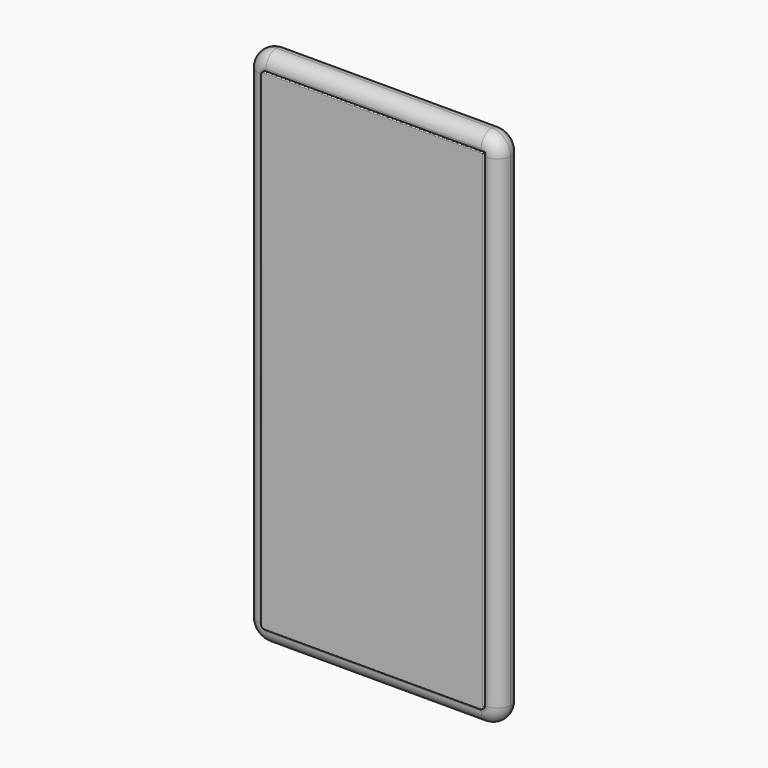
from build123d import *

# Parameters (mm, degrees)
F0_W     = 67
F0_H     = 138
F1_DEPTH = 6.9
F2_R     = 5
F3_R     = 3.44999
F6_DEPTH = 0.5
F7_R     = 0.25


# Not quite as in the source:
# - a fillet or chamfer is up to 0.001 mm smaller than in the source, because OpenCascade refuses the exact size


with BuildPart() as f1:
    # F0 (on Front) → F1 (new body)
    with BuildSketch(Plane.XZ):
        with Locations((33.5, 69)):
            Rectangle(F0_W, F0_H)
    extrude(amount=-F1_DEPTH)

    # F2
    f2_edges = [f1.edges().sort_by_distance(p)[0] for p in [
        (67, 3.45, 138),
        (67, 3.45, 0),
        (0, 3.45, 138),
        (0, 3.45, 0),
    ]]
    fillet(f2_edges, radius=F2_R)

    # F3 (radius 3.45 in the source; OpenCascade refuses exactly that, so slightly less here)
    f3_edges = [f1.edges().sort_by_distance(p)[0] for p in [
        (67, 0, 69),
        (0, 6.9, 69),
        (1.464466, 6.9, 136.535534),
        (1.464466, 6.9, 1.464466),
        (33.5, 6.9, 138),
        (33.5, 6.9, 0),
        (65.535534, 6.9, 136.535534),
        (65.535534, 6.9, 1.464466),
        (67, 6.9, 69),
    ]]
    fillet(f3_edges, radius=F3_R)

    # F5 (on face) → F6 (join)
    with BuildSketch(Plane.XZ):
        with BuildLine():
            ThreePointArc((5, 134.05), (4.2575378798, 133.7424621202), (3.95, 133))
            Line((3.95, 133), (3.95, 5))
            ThreePointArc((3.95, 5), (4.2575378798, 4.2575378798), (5, 3.95))
            Line((5, 3.95), (62, 3.95))
            ThreePointArc((62, 3.95), (62.7424621202, 4.2575378798), (63.05, 5))
            Line((63.05, 5), (63.05, 134.05))
            Line((63.05, 134.05), (5, 134.05))
        make_face()
    extrude(amount=F6_DEPTH)

    # F7
    f7_edges = [f1.edges().sort_by_distance(p)[0] for p in [
        (3.95, -0.5, 69),
    ]]
    fillet(f7_edges, radius=F7_R)


solid = f1.part
